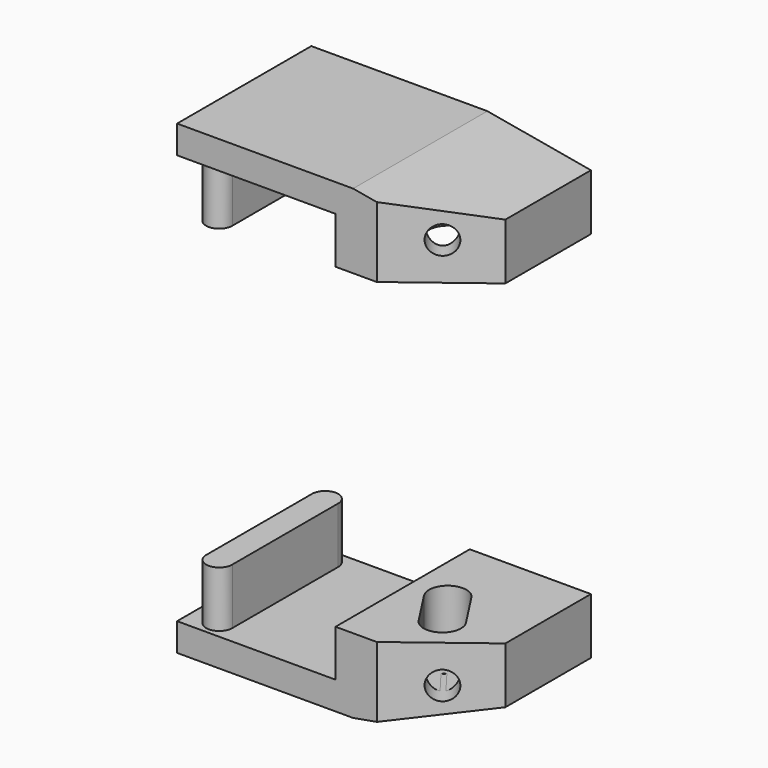
from build123d import *

# Parameters (mm, degrees)
F0_W      = 30
F0_H      = 18
F1_DEPTH  = 9
F2_W      = 30
F2_H      = 18
F3_DEPTH  = 6
F5_DEPTH  = 25
F7_DEPTH  = 5
F8_R      = 1.5
F9_DEPTH  = 5
F11_DEPTH = 5.52
F13_DEPTH = 25


with BuildPart() as f1:
    # F0 (on Top) → F1 (new body)
    with BuildSketch(Plane.XY):
        with Locations((15, -9)):
            Rectangle(F0_W, F0_H)
    extrude(amount=F1_DEPTH)

    # F2 (on face) → F3 (cut)
    with BuildSketch(Plane.XY.offset(9)):
        with Locations((15, -9)):
            Rectangle(F2_W, F2_H)
        with BuildLine():
            ThreePointArc((1.6, -1.9), (3, -0.5), (4.4, -1.9))
            Line((4.4, -1.9), (4.4, -16.1))
            ThreePointArc((4.4, -16.1), (3, -17.5), (1.6, -16.1))
            Line((1.6, -16.1), (1.6, -1.9))
        make_face(mode=Mode.SUBTRACT)
    extrude(amount=-F3_DEPTH, mode=Mode.SUBTRACT)

    # F4 (on face) → F5 (cut)
    with BuildSketch(Plane.XY.offset(3)):
        Polygon((30, -11.476942338), (21.424215287, -18), (30, -18), align=None)
    extrude(amount=-F5_DEPTH, mode=Mode.SUBTRACT)

    # F6 (on face) → F7 (join)
    with BuildSketch(Plane.XY.offset(3)):
        Polygon((30, -11.476942338), (30, 0), (17, 0), (17, -11.476942338), (17, -18), (21.424215287, -18), align=None)
    extrude(amount=F7_DEPTH)

    # F8 (on face) → F9 (cut)
    with BuildSketch(Plane(origin=(16.5256296321, -21.7260446429, 0), x_dir=(0.7959179518, 0.6054045044, 0), z_dir=(0.6054045044, -0.7959179518, 0))):
        with Locations((11.6600664333, 3.9596073329)):
            Circle(F8_R)
    extrude(amount=-F9_DEPTH, mode=Mode.SUBTRACT)

    # F10 (on face) → F11 (cut)
    with BuildSketch(Plane.XY.offset(8)):
        with BuildLine():
            Line((19.254878048, -8.9549584287), (21.8133040316, -12.8929519365))
            ThreePointArc((21.8133040316, -12.8929519365), (24.6189354383, -13.2459612648), (24.9732833017, -10.4404985993))
            Line((24.9732833017, -10.4404985993), (22.4684233059, -6.584955205))
            ThreePointArc((22.4684233059, -6.584955205), (19.7449236449, -6.2557593582), (19.254878048, -8.9549584287))
        make_face()
    extrude(amount=-F11_DEPTH, mode=Mode.SUBTRACT)

    # F12 (on face) → F13 (cut)
    with BuildSketch(Plane(origin=(0, 0, 0), x_dir=(-1, 0, 0), z_dir=(0, 1, 0))):
        Polygon((-18.8889801502, 0), (-30, 1.9705295563), (-30, 0), align=None)
    extrude(amount=-F13_DEPTH, mode=Mode.SUBTRACT)


with BuildPart() as f15_1:
    # F15: instance of F1
    add(f1.part.mirror(Plane.XY.offset(25)))


solid = Compound([f1.part, f15_1.part])
